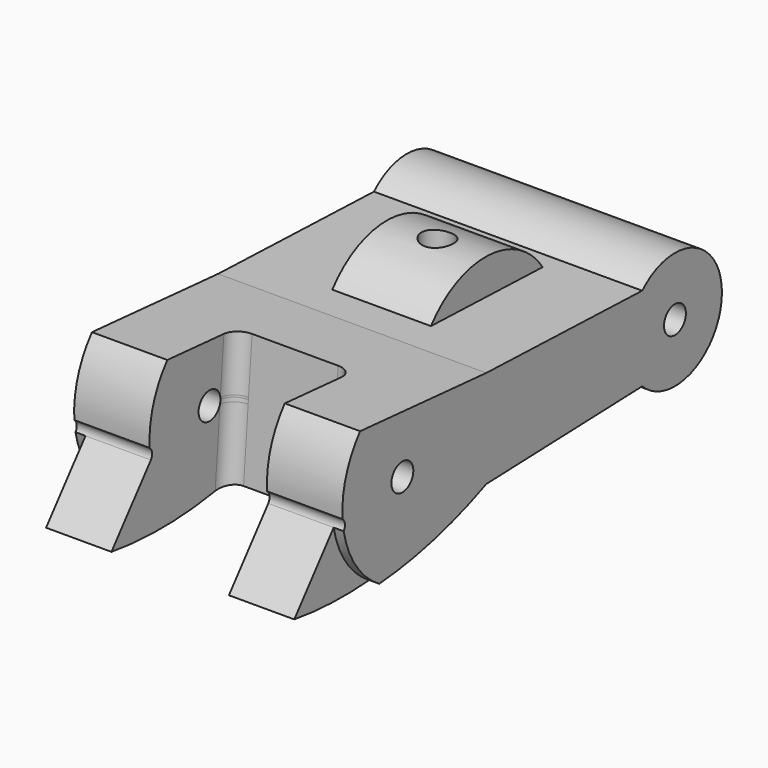
from build123d import *

# Parameters (mm, degrees)
F0_R      = 4.445
F1_DEPTH  = 43.5102
F4_DEPTH  = 16.002
F5_R      = 5.08
F6_DEPTH  = 76.2
F8_DEPTH  = 3.2512
F10_DEPTH = 48.8043176288
F11_R     = 5.08


# Not quite as in the source:
# - a pattern or mirror of a feature is missing from the dataset's text; its kind, count and spacing are read off the source's solid


with BuildPart() as f1:
    # F0 (on Right) → F1 (new body, symmetric)
    with BuildSketch(Plane.YZ):
        with BuildLine():
            Line((-20.0435682294, -15.8600244388), (43.1716607283, -13.6525))
            ThreePointArc((43.1716607283, -13.6525), (75.5074329584, 0), (43.1716607283, 13.6525))
            Line((43.1716607283, 13.6525), (-20.0435682294, 15.8600244388))
            ThreePointArc((-20.0435682294, 15.8600244388), (-15.7347770092, 0), (-20.0435682294, -15.8600244388))
        make_face()
        with Locations((56.4574329584, 0)):
            Circle(F0_R, mode=Mode.SUBTRACT)
        with BuildLine():
            ThreePointArc((-93.8586293632, -25.5824005626), (-56.2599595636, -25.9685392928), (-20.0435682294, -15.8600244388))
            ThreePointArc((-20.0435682294, -15.8600244388), (-15.7347770092, 0), (-20.0435682294, 15.8600244388))
            Line((-20.0435682294, 15.8600244388), (-71.2014077133, 20.0125123513))
            ThreePointArc((-71.2014077133, 20.0125123513), (-76.9181304267, 9.5922039668), (-78.3441527071, -2.2073810202))
            ThreePointArc((-78.3441527071, -2.2073810202), (-77.3808721828, -3.9314055649), (-77.8723212002, -5.8441647924))
            Line((-77.8723212002, -5.8441647924), (-93.8586293632, -25.5824005626))
        make_face()
        with Locations((-54.0887770092, 0)):
            Circle(F0_R, mode=Mode.SUBTRACT)
    extrude(amount=F1_DEPTH, both=True)

    # F3 (on Right) → F4 (join, symmetric)
    with BuildSketch(Plane.YZ):
        with BuildLine():
            ThreePointArc((37.2042329584, 13.8608871696), (14.9518760887, 26.202001098), (-8.1071477478, 15.4431954506))
            Line((-8.1071477478, 15.4431954506), (37.2042329584, 13.8608871696))
        make_face()
    extrude(amount=F4_DEPTH, both=True)

    # F5 (on Top) → F6 (cut, symmetric)
    with BuildSketch(Plane.XY):
        with Locations((0, 14.5474329584)):
            Circle(F5_R)
    extrude(amount=F6_DEPTH, both=True, mode=Mode.SUBTRACT)

    # F7 (on face) → F8 (cut)
    with BuildSketch(Plane.YZ.offset(43.5102)):
        with BuildLine():
            ThreePointArc((-63.4642960228, -26.7193360516), (-72.8742694492, -17.8043026874), (-77.8723212002, -5.8441647924))
            Line((-77.8723212002, -5.8441647924), (-93.8586293632, -25.5824005626))
            ThreePointArc((-93.8586293632, -25.5824005626), (-78.69393168, -27.0188799259), (-63.4642960228, -26.7193360516))
        make_face()
    f8 = extrude(amount=-F8_DEPTH, mode=Mode.SUBTRACT)

    # F8_copies: F8 across plane
    add(f8.mirror(Plane(origin=(0, 0, 0), x_dir=(0, 0, -1), z_dir=(-1, 0, 0))), mode=Mode.SUBTRACT)

    # F9 (on face) → F10 (cut, through all)
    with BuildSketch(Plane(origin=(0, 1.1477392706, 14.1399234898), x_dir=(1, 0, 0), z_dir=(0, 0.0809040348, 0.9967218956))):
        Polygon((19.05, -91.4812315527), (19.05, -44.4912315527), (0, -44.4912315527), (-19.05, -44.4912315527), (-19.05, -91.4812315527), align=None)
    extrude(amount=-F10_DEPTH, mode=Mode.SUBTRACT)

    # F11
    f11_edges = [f1.edges().sort_by_distance(p)[0] for p in [
        (19.05, -44.905298, -3.298502),
        (-19.05, -44.905298, -3.298502),
    ]]
    fillet(f11_edges, radius=F11_R)


solid = f1.part
